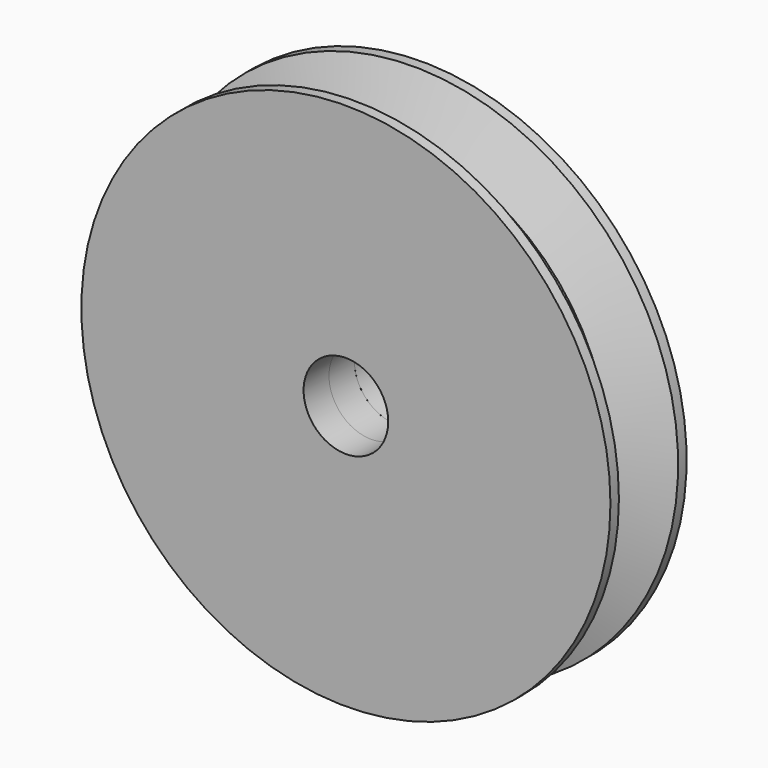
from build123d import *

# Parameters (mm, degrees)
F0_R       = 20
F0_R_2     = 4
F1_DEPTH   = 3
F2_R       = 25
F2_R_2     = 20
F2_R_3     = 4
F3_DEPTH   = 3
F4_R       = 25
F4_R_2     = 20
F4_R_3     = 4
F5_DEPTH   = 3
F6_SIZE2   = 5
F6_SIZE    = 2
F6_2_SIZE2 = 5
F6_2_SIZE  = 2


with BuildPart() as f1:
    # F0 (on Front) → F1 (new body)
    with BuildSketch(Plane.XZ):
        Circle(F0_R)
        Circle(F0_R_2, mode=Mode.SUBTRACT)
    extrude(amount=F1_DEPTH)


with BuildPart() as f3:
    # F2 (on face) → F3 (new body)
    with BuildSketch(Plane(origin=(0, 0, 0), x_dir=(-1, 0, 0), z_dir=(0, 1, 0))):
        Circle(F2_R)
        Circle(F2_R_2, mode=Mode.SUBTRACT)
        Circle(F2_R_2)
        Circle(F2_R_3, mode=Mode.SUBTRACT)
    extrude(amount=F3_DEPTH)

    # F6
    f6_edges = [f3.edges().sort_by_distance(p)[0] for p in [
        (25, 0, 0),
    ]]
    f6_side = f3.faces().sort_by_distance((25, 1.5, 0))[0]
    chamfer(f6_edges, length=F6_SIZE, length2=F6_SIZE2, reference=f6_side)


with BuildPart() as f5:
    # F4 (on face) → F5 (new body)
    with BuildSketch(Plane.XZ.offset(3)):
        Circle(F4_R)
        Circle(F4_R_2, mode=Mode.SUBTRACT)
        Circle(F4_R_2)
        Circle(F4_R_3, mode=Mode.SUBTRACT)
    extrude(amount=F5_DEPTH)

    # F6#2
    f6_2_edges = [f5.edges().sort_by_distance(p)[0] for p in [
        (-25, -3, 0),
    ]]
    f6_2_side = f5.faces().sort_by_distance((-25, -4.5, 0))[0]
    chamfer(f6_2_edges, length=F6_2_SIZE, length2=F6_2_SIZE2, reference=f6_2_side)


solid = Compound([f1.part, f3.part, f5.part])
